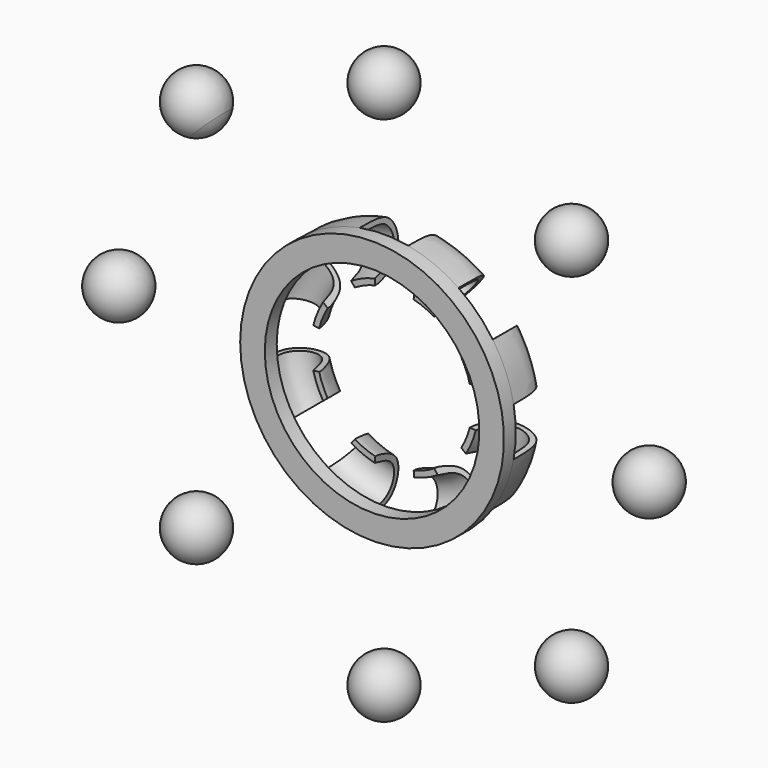
from build123d import *

# Parameters (mm, degrees)
F4_DEPTH = 10


# Not quite as in the source:
# - a feature names something its author has since deleted; it is built from what else it names


with BuildPart() as f3:
    # F2 (on Top) → F3 (revolve)
    with BuildSketch(Plane.XY):
        with BuildLine():
            add(Edge.make_bspline(
                [(-14.5997647196, 0), (-14.5914583176, 1.0201638138), (-14.6125249315, 2.8173851501), (-13.8683408491, 4.3344980804), (-11.9931970887, 5.1910127795), (-9.43948285, 4.691257471), (-8.6999247521, 2.1806928113), (-8.6007463336, 1.8402322465), (-8.6007463336, 1.4504397096)],
                knots=[0, 0, 0, 0, 0.2043736541, 0.3547086736, 0.521989101, 0.708044694, 0.8897773391, 1, 1, 1, 1], degree=3))
            add(Edge.make_bspline(
                [(-14.6007463336, -1.65), (-14.6055433257, -1.2194524819), (-14.597283957, -0.5071059674), (-14.6032171324, -0.1503027161), (-14.5997647196, 0)],
                knots=[0, 0, 0, 0, 0.6079019082, 1, 1, 1, 1], degree=3))
            Line((-14.6007463336, -1.65), (-11.8757463336, -1.65))
            Line((-11.8757463336, -1.65), (-11.8757463336, 0))
            Line((-11.8757463336, 0), (-14.002260752, 0))
            add(Edge.make_bspline(
                [(-9.2507463336, 1.4504397096), (-9.2948862872, 1.6229423508), (-9.3948133712, 2.0867211392), (-9.898911746, 4.1097579941), (-11.9854122258, 4.611211307), (-13.4616431973, 3.7705932324), (-13.9889094664, 2.6159317193), (-14.002559664, 1.02456396), (-14.002260752, 0)],
                knots=[0, 0, 0, 0, 0.1060992717, 0.2899537281, 0.4734473247, 0.6392405331, 0.7826134695, 1, 1, 1, 1], degree=3))
            Line((-9.2507463336, 1.4504397096), (-8.6007463336, 1.4504397096))
        make_face()
    revolve(axis=Axis((0, 0.8276371518, 0), (0, 1, 0)))

    # F1 (on Front) → F4 (cut)
    with BuildSketch(Plane.XZ):
        Polygon((-5.913569041, -1.9002265742), (-5.913569041, 0), (-14.8067781538, 0), (-14.8067781538, -2.725), align=None)
        Polygon((-14.8067781538, 0), (-5.913569041, 0), (-5.913569041, 1.9002265742), (-14.8067781538, 2.725), align=None)
        Polygon((-5.5251878663, 2.8378616735), (-4.1815247699, 4.1815247699), (-10.4699732401, 10.4699732401), (-12.3968392188, 8.5431072614), align=None)
        Polygon((-10.4699732401, 10.4699732401), (-4.1815247699, 4.1815247699), (-2.8378616735, 5.5251878663), (-8.5431072614, 12.3968392188), align=None)
        Polygon((2.8378616735, 5.5251878663), (4.1815247699, 4.1815247699), (10.4699732401, 10.4699732401), (8.5431072614, 12.3968392188), align=None)
        Polygon((10.4699732401, 10.4699732401), (4.1815247699, 4.1815247699), (5.5251878663, 2.8378616735), (12.3968392188, 8.5431072614), align=None)
        Polygon((5.913569041, 1.9002265742), (5.913569041, 0), (14.8067781538, 0), (14.8067781538, 2.725), align=None)
        Polygon((14.8067781538, 0), (5.913569041, 0), (5.913569041, -1.9002265742), (14.8067781538, -2.725), align=None)
        Polygon((-2.8378616735, -5.5251878663), (-4.1815247699, -4.1815247699), (-10.4699732401, -10.4699732401), (-8.5431072614, -12.3968392188), align=None)
        Polygon((-10.4699732401, -10.4699732401), (-4.1815247699, -4.1815247699), (-5.5251878663, -2.8378616735), (-12.3968392188, -8.5431072614), align=None)
        Polygon((5.5251878663, -2.8378616735), (4.1815247699, -4.1815247699), (10.4699732401, -10.4699732401), (12.3968392188, -8.5431072614), align=None)
        Polygon((10.4699732401, -10.4699732401), (4.1815247699, -4.1815247699), (2.8378616735, -5.5251878663), (8.5431072614, -12.3968392188), align=None)
        Polygon((1.9002265742, -5.913569041), (0, -5.913569041), (0, -14.8067781538), (2.725, -14.8067781538), align=None)
        Polygon((0, -14.8067781538), (0, -5.913569041), (-1.9002265742, -5.913569041), (-2.725, -14.8067781538), align=None)
        Polygon((1.9002265742, 5.913569041), (2.725, 14.8067781538), (-2.725, 14.8067781538), (-1.9002265742, 5.913569041), align=None)
    extrude(amount=-F4_DEPTH, mode=Mode.SUBTRACT)


with BuildPart() as f6:
    # F5 (on Front) → F6 (revolve)
    with BuildSketch(Plane.XZ):
        with BuildLine():
            Line((18.5119370005, 18.5119370005), (23.0020650611, 23.0020650611))
            ThreePointArc((23.0020650611, 23.0020650611), (18.5119370005, 23.0020650611), (18.5119370005, 18.5119370005))
        make_face()
    revolve(axis=Axis((20.7570010308, 0, 20.7570010308), (-0.7071067812, 0, -0.7071067812)))


with BuildPart() as f7:
    # F5 (on Front) → F7 (revolve)
    with BuildSketch(Plane.XZ):
        with BuildLine():
            Line((0, 26.1798323719), (0, 32.5298323719))
            ThreePointArc((0, 32.5298323719), (-3.175, 29.3548323719), (0, 26.1798323719))
        make_face()
    revolve(axis=Axis((0, 0, 29.3548323719), (0, 0, -1)))


with BuildPart() as f8:
    # F5 (on Front) → F8 (revolve)
    with BuildSketch(Plane.XZ):
        with BuildLine():
            ThreePointArc((-18.5119370005, 18.5119370005), (-17.8236835151, 19.541981133), (-17.5820010308, 20.7570010308))
            ThreePointArc((-17.5820010308, 20.7570010308), (-19.541981133, 23.6903185465), (-23.0020650611, 23.0020650611))
            Line((-23.0020650611, 23.0020650611), (-18.5119370005, 18.5119370005))
        make_face()
    revolve(axis=Axis((-20.7570010308, 0, 20.7570010308), (0.7071067812, 0, -0.7071067812)))


with BuildPart() as f9:
    # F5 (on Front) → F9 (revolve)
    with BuildSketch(Plane.XZ):
        with BuildLine():
            Line((-32.5298323719, 0), (-26.1798323719, 0))
            ThreePointArc((-26.1798323719, 0), (-29.3548323719, 3.175), (-32.5298323719, 0))
        make_face()
    revolve(axis=Axis((-29.3548323719, 0, 0), (1, 0, 0)))


with BuildPart() as f10:
    # F5 (on Front) → F10 (revolve)
    with BuildSketch(Plane.XZ):
        with BuildLine():
            Line((-23.0020650611, -23.0020650611), (-18.5119370005, -18.5119370005))
            ThreePointArc((-18.5119370005, -18.5119370005), (-23.0020650611, -18.5119370005), (-23.0020650611, -23.0020650611))
        make_face()
    revolve(axis=Axis((-20.7570010308, 0, -20.7570010308), (0.7071067812, 0, 0.7071067812)))


with BuildPart() as f11:
    # F5 (on Front) → F11 (revolve)
    with BuildSketch(Plane.XZ):
        with BuildLine():
            Line((0, -32.5298323719), (0, -26.1798323719))
            ThreePointArc((0, -26.1798323719), (-3.175, -29.3548323719), (0, -32.5298323719))
        make_face()
    revolve(axis=Axis((0, 0, -29.3548323719), (0, 0, 1)))


with BuildPart() as f12:
    # F5 (on Front) → F12 (revolve)
    with BuildSketch(Plane.XZ):
        with BuildLine():
            Line((26.1798323719, 0), (32.5298323719, 0))
            ThreePointArc((32.5298323719, 0), (29.3548323719, 3.175), (26.1798323719, 0))
        make_face()
    revolve(axis=Axis((29.3548323719, 0, 0), (-1, 0, 0)))


with BuildPart() as f13:
    # F5 (on Front) → F13 (revolve)
    with BuildSketch(Plane.XZ):
        with BuildLine():
            ThreePointArc((18.5119370005, -18.5119370005), (18.5119370005, -23.0020650611), (23.0020650611, -23.0020650611))
            Line((23.0020650611, -23.0020650611), (18.5119370005, -18.5119370005))
        make_face()
    revolve(axis=Axis((20.7570010308, 0, -20.7570010308), (-0.7071067812, 0, 0.7071067812)))


solid = Compound([f3.part, f6.part, f7.part, f8.part, f9.part, f10.part, f11.part, f12.part, f13.part])
